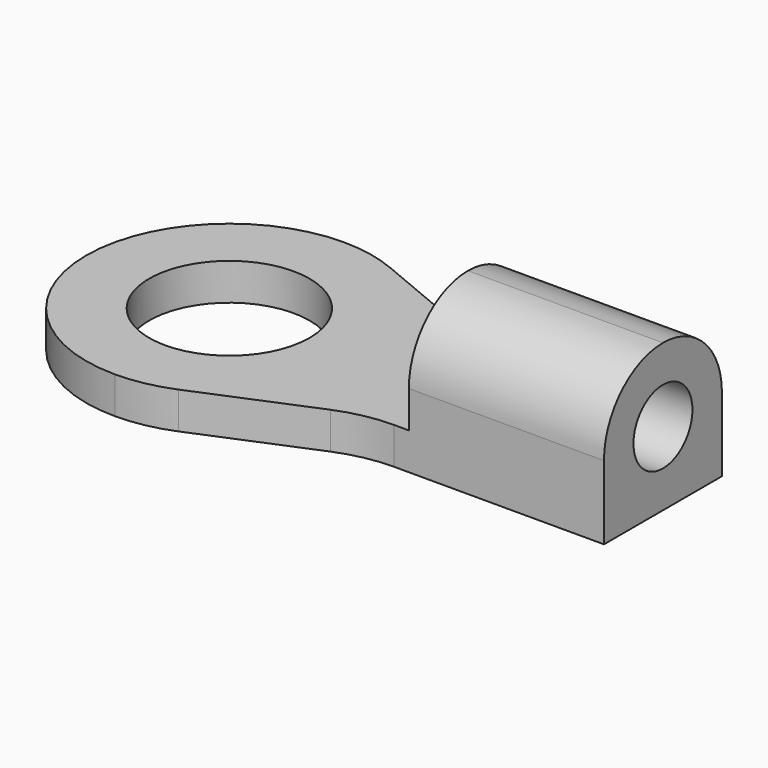
from build123d import *

# Parameters (mm, degrees)
F0_R     = 1.85
F1_DEPTH = 0.85
F2_W     = 4.5
F2_H     = 3.4
F3_DEPTH = 2.55
F4_R     = 1.69999
F5_R     = 0.85
F6_DEPTH = 25


# Not quite as in the source:
# - a fillet or chamfer is up to 0.001 mm smaller than in the source, because OpenCascade refuses the exact size


with BuildPart() as f1:
    # F0 (on Top) → F1 (new body)
    with BuildSketch(Plane.XY):
        with BuildLine():
            Line((8.46, 1.6), (13.3, 1.6))
            Line((13.3, 1.6), (13.3, 5))
            Line((13.3, 5), (8.46, 5))
            ThreePointArc((8.46, 5), (7.812816754, 5.0640837702), (7.1907692308, 5.2538461538))
            Line((7.1907692308, 5.2538461538), (4.5692307692, 6.3461538462))
            ThreePointArc((4.5692307692, 6.3461538462), (3.947183246, 6.5359162298), (3.3, 6.6))
            ThreePointArc((3.3, 6.6), (0.9665476221, 5.6334523779), (0, 3.3))
            ThreePointArc((0, 3.3), (0.9665476221, 0.9665476221), (3.3, 0))
            ThreePointArc((3.3, 0), (3.947183246, 0.0640837702), (4.5692307692, 0.2538461538))
            Line((4.5692307692, 0.2538461538), (7.1907692308, 1.3461538462))
            ThreePointArc((7.1907692308, 1.3461538462), (7.812816754, 1.5359162298), (8.46, 1.6))
        make_face()
        with Locations((3.3, 3.3)):
            Circle(F0_R, mode=Mode.SUBTRACT)
    extrude(amount=F1_DEPTH)

    # F2 (on face) → F3 (join)
    with BuildSketch(Plane.XY.offset(0.85)):
        with Locations((11.05, 3.3)):
            Rectangle(F2_W, F2_H)
    extrude(amount=F3_DEPTH)

    # F4 (radius 1.7 in the source; OpenCascade refuses exactly that, so slightly less here)
    f4_edges = [f1.edges().sort_by_distance(p)[0] for p in [
        (11.05, 5, 3.4),
        (11.05, 1.6, 3.4),
    ]]
    fillet(f4_edges, radius=F4_R)

    # F5 (on face) → F6 (cut)
    with BuildSketch(Plane.YZ.offset(13.3)):
        with Locations((3.3, 1.7)):
            Circle(F5_R)
    extrude(amount=-F6_DEPTH, mode=Mode.SUBTRACT)


solid = f1.part
